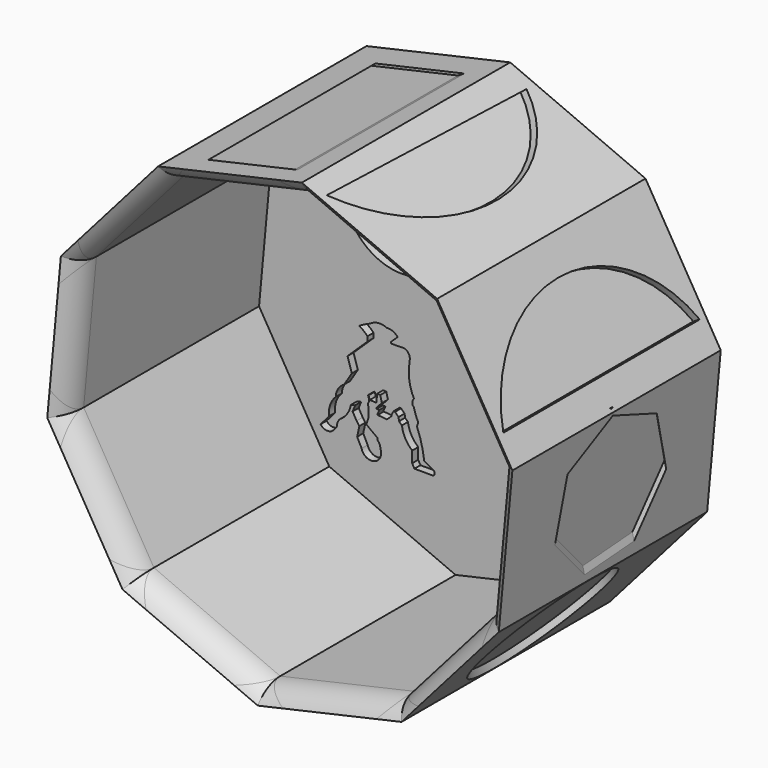
from build123d import *

# Parameters (mm, degrees)
F1_DEPTH      = 25.4
F1_DEPTH_BACK = 12.7
F2_DEPTH      = 19.05
F3_T          = -2.54
F4_T4_DEPTH   = 48.5082887961
F4_T10_DEPTH  = 48.5082887961
F4_T16_DEPTH  = 48.5082887961
F4_T22_DEPTH  = 48.5082887961
F4_T28_DEPTH  = 48.5082887961
F4_T34_DEPTH  = 48.5082887961
F4_T40_DEPTH  = 48.5082887961
F4_T46_DEPTH  = 48.5082887961
F4_T52_DEPTH  = 48.5082887961
F4_T58_DEPTH  = 48.5082887961
F4_T65_DEPTH  = 48.5082887961
F4_T71_DEPTH  = 48.5082887961
F4_T80_DEPTH  = 48.5082887961
F4_T86_DEPTH  = 48.5082887961
F4_T95_DEPTH  = 48.5082887961
F4_T101_DEPTH = 48.5082887961
F4_T110_DEPTH = 48.5082887961
F4_T116_DEPTH = 48.5082887961
F4_T125_DEPTH = 48.5082887961
F4_T131_DEPTH = 48.5082887961
F4_T140_DEPTH = 48.5082887961
F4_T146_DEPTH = 48.5082887961
F4_T155_DEPTH = 48.5082887961
F4_T161_DEPTH = 48.5082887961
F4_T170_DEPTH = 48.5082887961
F4_T176_DEPTH = 48.5082887961
F4_T185_DEPTH = 48.5082887961
F4_T191_DEPTH = 48.5082887961
F4_T200_DEPTH = 48.5082887961
F4_T206_DEPTH = 48.5082887961
F5_R          = 9.7214330453
F5_R_2        = 9.651520044
F6_DEPTH      = 1.27
F8_R          = 12.2677315005
F17_DEPTH     = 1.27
F12_W         = 15.3330643661
F12_H         = 35.0531535223
F18_DEPTH     = 1.27
F19_DEPTH     = 1.27


# Not quite as in the source:
# - a fillet or chamfer that OpenCascade refuses, or shapes differently, is made with other operations: its cross-section is extruded or revolved along the edge and cut away or added


with BuildPart() as f1:
    # F0 (on Front) → F1 (new body, two sides)
    with BuildSketch(Plane.XZ) as f1_sk:
        Polygon((26.439509189, 30.0967257209), (3.6996007358, 39.8895161624), (-20.4534294537, 34.4458672246), (-36.7939447783, 15.845067779), (-39.0804237778, -8.8080090041), (-26.439509189, -30.0967257209), (-3.6996007358, -39.8895161624), (20.4534294537, -34.4458672246), (36.7939447783, -15.845067779), (39.0804237778, 8.8080090041), align=None)
    extrude(amount=F1_DEPTH)
    extrude(f1_sk.sketch, amount=-F1_DEPTH_BACK)

    # F0 (on Front) → F2 (join)
    with BuildSketch(Plane.XZ):
        Polygon((26.439509189, 30.0967257209), (3.6996007358, 39.8895161624), (-20.4534294537, 34.4458672246), (-36.7939447783, 15.845067779), (-39.0804237778, -8.8080090041), (-26.439509189, -30.0967257209), (-3.6996007358, -39.8895161624), (20.4534294537, -34.4458672246), (36.7939447783, -15.845067779), (39.0804237778, 8.8080090041), align=None)
    extrude(amount=-F2_DEPTH)

    # F3
    f3_openings = [f1.faces().sort_by_distance(p)[0] for p in [
        (0, -25.4, 0),
    ]]
    offset(amount=F3_T, openings=f3_openings)

    # F4: fillet of radius 5.08 on 10 edges, made by hand


with BuildPart() as f4_tool2:
    # F4_s3 → F4_t4 (new body)
    with BuildSketch(Plane(origin=(12.383215929, 0, -20.8547232956), x_dir=(0, 1, 0), z_dir=(-0.5105608232, 0, 0.85984164))):
        with BuildLine():
            ThreePointArc((-25.4, -40.64), (-23.9121024484, -37.0478975516), (-20.32, -35.56))
            Line((-20.32, -35.56), (-25.4, -35.56))
            Line((-25.4, -35.56), (-25.4, -40.64))
        make_face()
    extrude(amount=F4_T4_DEPTH)

    split(bisect_by=Plane(origin=(35.4080386595, 0, -3.2839607616), x_dir=(0, 1, 0), z_dir=(-0.9957266215, 0, 0.0923498527)), keep=Keep.TOP)

    split(bisect_by=Plane(origin=(14.0649179649, 0, 32.6602462122), x_dir=(0, 1, 0), z_dir=(-0.395526377, 0, -0.9184546179)), keep=Keep.TOP)


with BuildPart() as f1_1:
    add(f1.part)

    # F4_t1: cut F4_tool2
    add(f4_tool2.part, mode=Mode.SUBTRACT)


with BuildPart() as f4_tool8:
    # F4_s9 → F4_t10 (new body)
    with BuildSketch(Plane(origin=(-2.2398666623, 0, -24.1504972582), x_dir=(0, 1, 0), z_dir=(0.0923498527, 0, 0.9957266215))):
        with BuildLine():
            ThreePointArc((-25.4, -40.64), (-23.9121024484, -37.0478975516), (-20.32, -35.56))
            Line((-20.32, -35.56), (-25.4, -35.56))
            Line((-25.4, -35.56), (-25.4, -40.64))
        make_face()
    extrude(amount=F4_T10_DEPTH)

    split(bisect_by=Plane(origin=(30.5759687179, 0, 18.1555428717), x_dir=(0, 1, 0), z_dir=(-0.85984164, 0, -0.5105608232)), keep=Keep.TOP)

    split(bisect_by=Plane(origin=(26.7154413083, 0, -23.4691030017), x_dir=(0, 1, 0), z_dir=(-0.7512778771, 0, 0.6599860237)), keep=Keep.TOP)


with BuildPart() as f1_2:
    add(f1_1.part)

    # F4_t7: cut F4_tool8
    add(f4_tool8.part, mode=Mode.SUBTRACT)


with BuildPart() as f4_tool14:
    # F4_s15 → F4_t16 (new body)
    with BuildSketch(Plane(origin=(-16.0073963188, 0, -18.2216021133), x_dir=(0, 1, 0), z_dir=(0.6599860237, 0, 0.7512778771))):
        with BuildLine():
            ThreePointArc((-25.4, -40.64), (-23.9121024484, -37.0478975516), (-20.32, -35.56))
            Line((-20.32, -35.56), (-25.4, -35.56))
            Line((-25.4, -35.56), (-25.4, -40.64))
        make_face()
    extrude(amount=F4_T16_DEPTH)

    split(bisect_by=Plane(origin=(35.4080386595, 0, -3.2839607616), x_dir=(0, 1, 0), z_dir=(-0.9957266215, 0, 0.0923498527)), keep=Keep.TOP)

    split(bisect_by=Plane(origin=(7.8184534017, 0, -34.6898455806), x_dir=(0, 1, 0), z_dir=(-0.2198665186, 0, 0.9755299657)), keep=Keep.TOP)


with BuildPart() as f1_3:
    add(f1_2.part)

    # F4_t13: cut F4_tool14
    add(f4_tool14.part, mode=Mode.SUBTRACT)


with BuildPart() as f4_tool20:
    # F4_s21 → F4_t22 (new body)
    with BuildSketch(Plane(origin=(-23.6606446529, 0, -5.3326742906), x_dir=(0, 1, 0), z_dir=(0.9755299657, 0, 0.2198665186))):
        with BuildLine():
            ThreePointArc((-25.4, -40.64), (-23.9121024484, -37.0478975516), (-20.32, -35.56))
            Line((-20.32, -35.56), (-25.4, -35.56))
            Line((-25.4, -35.56), (-25.4, -40.64))
        make_face()
    extrude(amount=F4_T22_DEPTH)

    split(bisect_by=Plane(origin=(-14.0649179649, 0, -32.6602462122), x_dir=(0, 1, 0), z_dir=(0.395526377, 0, 0.9184546179)), keep=Keep.TOP)

    split(bisect_by=Plane(origin=(26.7154413083, 0, -23.4691030017), x_dir=(0, 1, 0), z_dir=(-0.7512778771, 0, 0.6599860237)), keep=Keep.TOP)


with BuildPart() as f1_4:
    add(f1_3.part)

    # F4_t19: cut F4_tool20
    add(f4_tool20.part, mode=Mode.SUBTRACT)


with BuildPart() as f4_tool26:
    # F4_s27 → F4_t28 (new body)
    with BuildSketch(Plane(origin=(-22.2763309254, 0, 9.5931538602), x_dir=(0, 1, 0), z_dir=(0.9184546179, 0, -0.395526377))):
        with BuildLine():
            ThreePointArc((-25.4, -40.64), (-23.9121024484, -37.0478975516), (-20.32, -35.56))
            Line((-20.32, -35.56), (-25.4, -35.56))
            Line((-25.4, -35.56), (-25.4, -40.64))
        make_face()
    extrude(amount=F4_T28_DEPTH)

    split(bisect_by=Plane(origin=(-30.5759687179, 0, -18.1555428717), x_dir=(0, 1, 0), z_dir=(0.85984164, 0, 0.5105608232)), keep=Keep.TOP)

    split(bisect_by=Plane(origin=(7.8184534017, 0, -34.6898455806), x_dir=(0, 1, 0), z_dir=(-0.2198665186, 0, 0.9755299657)), keep=Keep.TOP)


with BuildPart() as f1_5:
    add(f1_4.part)

    # F4_t25: cut F4_tool26
    add(f4_tool26.part, mode=Mode.SUBTRACT)


with BuildPart() as f4_tool32:
    # F4_s33 → F4_t34 (new body)
    with BuildSketch(Plane(origin=(22.2763309254, 0, -9.5931538602), x_dir=(0, 1, 0), z_dir=(-0.9184546179, 0, 0.395526377))):
        with BuildLine():
            ThreePointArc((-25.4, -40.64), (-23.9121024484, -37.0478975516), (-20.32, -35.56))
            Line((-20.32, -35.56), (-25.4, -35.56))
            Line((-25.4, -35.56), (-25.4, -40.64))
        make_face()
    extrude(amount=F4_T34_DEPTH)

    split(bisect_by=Plane(origin=(30.5759687179, 0, 18.1555428717), x_dir=(0, 1, 0), z_dir=(-0.85984164, 0, -0.5105608232)), keep=Keep.TOP)

    split(bisect_by=Plane(origin=(-7.8184534017, 0, 34.6898455806), x_dir=(0, 1, 0), z_dir=(0.2198665186, 0, -0.9755299657)), keep=Keep.TOP)


with BuildPart() as f1_6:
    add(f1_5.part)

    # F4_t31: cut F4_tool32
    add(f4_tool32.part, mode=Mode.SUBTRACT)


with BuildPart() as f4_tool38:
    # F4_s39 → F4_t40 (new body)
    with BuildSketch(Plane(origin=(23.6606446529, 0, 5.3326742906), x_dir=(0, 1, 0), z_dir=(-0.9755299657, 0, -0.2198665186))):
        with BuildLine():
            ThreePointArc((-25.4, -40.64), (-23.9121024484, -37.0478975516), (-20.32, -35.56))
            Line((-20.32, -35.56), (-25.4, -35.56))
            Line((-25.4, -35.56), (-25.4, -40.64))
        make_face()
    extrude(amount=F4_T40_DEPTH)

    split(bisect_by=Plane(origin=(14.0649179649, 0, 32.6602462122), x_dir=(0, 1, 0), z_dir=(-0.395526377, 0, -0.9184546179)), keep=Keep.TOP)

    split(bisect_by=Plane(origin=(-26.7154413083, 0, 23.4691030017), x_dir=(0, 1, 0), z_dir=(0.7512778771, 0, -0.6599860237)), keep=Keep.TOP)


with BuildPart() as f1_7:
    add(f1_6.part)

    # F4_t37: cut F4_tool38
    add(f4_tool38.part, mode=Mode.SUBTRACT)


with BuildPart() as f4_tool44:
    # F4_s45 → F4_t46 (new body)
    with BuildSketch(Plane(origin=(16.0073963188, 0, 18.2216021133), x_dir=(0, 1, 0), z_dir=(-0.6599860237, 0, -0.7512778771))):
        with BuildLine():
            ThreePointArc((-25.4, -40.64), (-23.9121024484, -37.0478975516), (-20.32, -35.56))
            Line((-20.32, -35.56), (-25.4, -35.56))
            Line((-25.4, -35.56), (-25.4, -40.64))
        make_face()
    extrude(amount=F4_T46_DEPTH)

    split(bisect_by=Plane(origin=(-7.8184534017, 0, 34.6898455806), x_dir=(0, 1, 0), z_dir=(0.2198665186, 0, -0.9755299657)), keep=Keep.TOP)

    split(bisect_by=Plane(origin=(-35.4080386595, 0, 3.2839607616), x_dir=(0, 1, 0), z_dir=(0.9957266215, 0, -0.0923498527)), keep=Keep.TOP)


with BuildPart() as f1_8:
    add(f1_7.part)

    # F4_t43: cut F4_tool44
    add(f4_tool44.part, mode=Mode.SUBTRACT)


with BuildPart() as f4_tool50:
    # F4_s51 → F4_t52 (new body)
    with BuildSketch(Plane(origin=(2.2398666623, 0, 24.1504972582), x_dir=(0, 1, 0), z_dir=(-0.0923498527, 0, -0.9957266215))):
        with BuildLine():
            ThreePointArc((-25.4, -40.64), (-23.9121024484, -37.0478975516), (-20.32, -35.56))
            Line((-20.32, -35.56), (-25.4, -35.56))
            Line((-25.4, -35.56), (-25.4, -40.64))
        make_face()
    extrude(amount=F4_T52_DEPTH)

    split(bisect_by=Plane(origin=(-26.7154413083, 0, 23.4691030017), x_dir=(0, 1, 0), z_dir=(0.7512778771, 0, -0.6599860237)), keep=Keep.TOP)

    split(bisect_by=Plane(origin=(-30.5759687179, 0, -18.1555428717), x_dir=(0, 1, 0), z_dir=(0.85984164, 0, 0.5105608232)), keep=Keep.TOP)


with BuildPart() as f1_9:
    add(f1_8.part)

    # F4_t49: cut F4_tool50
    add(f4_tool50.part, mode=Mode.SUBTRACT)


with BuildPart() as f4_tool56:
    # F4_s57 → F4_t58 (new body)
    with BuildSketch(Plane(origin=(-12.383215929, 0, 20.8547232956), x_dir=(0, 1, 0), z_dir=(0.5105608232, 0, -0.85984164))):
        with BuildLine():
            ThreePointArc((-25.4, -40.64), (-23.9121024484, -37.0478975516), (-20.32, -35.56))
            Line((-20.32, -35.56), (-25.4, -35.56))
            Line((-25.4, -35.56), (-25.4, -40.64))
        make_face()
    extrude(amount=F4_T58_DEPTH)

    split(bisect_by=Plane(origin=(-35.4080386595, 0, 3.2839607616), x_dir=(0, 1, 0), z_dir=(0.9957266215, 0, -0.0923498527)), keep=Keep.TOP)

    split(bisect_by=Plane(origin=(-14.0649179649, 0, -32.6602462122), x_dir=(0, 1, 0), z_dir=(0.395526377, 0, 0.9184546179)), keep=Keep.TOP)


with BuildPart() as f1_10:
    add(f1_9.part)

    # F4_t55: cut F4_tool56
    add(f4_tool56.part, mode=Mode.SUBTRACT)


with BuildPart() as f4_tool63:
    # F4_s64 → F4_t65 (new body)
    with BuildSketch(Plane(origin=(-2.2398666623, 0, -24.1504972582), x_dir=(0, 1, 0), z_dir=(0.0923498527, 0, 0.9957266215))):
        with BuildLine():
            ThreePointArc((-25.4, -40.64), (-23.9121024484, -37.0478975516), (-20.32, -35.56))
            Line((-20.32, -35.56), (-25.4, -35.56))
            Line((-25.4, -35.56), (-25.4, -40.64))
        make_face()
    extrude(amount=F4_T65_DEPTH)

    split(bisect_by=Plane(origin=(37.9371842781, 0, -3.5185293875), x_dir=(0, 1, 0), z_dir=(-0.9957266215, 0, 0.0923498527)), keep=Keep.TOP)

    split(bisect_by=Plane(origin=(32.7599664834, 0, 19.4523673625), x_dir=(0, 1, 0), z_dir=(-0.85984164, 0, -0.5105608232)), keep=Keep.TOP)

    split(bisect_by=Plane(origin=(30.5759687179, 0, 18.1555428717), x_dir=(0, 1, 0), z_dir=(0.85984164, 0, 0.5105608232)), keep=Keep.TOP)


with BuildPart() as f4_tool69:
    # F4_s70 → F4_t71 (new body)
    with BuildSketch(Plane(origin=(12.383215929, 0, -20.8547232956), x_dir=(0, 1, 0), z_dir=(-0.5105608232, 0, 0.85984164))):
        with BuildLine():
            ThreePointArc((-25.4, -40.64), (-23.9121024484, -37.0478975516), (-20.32, -35.56))
            Line((-20.32, -35.56), (-25.4, -35.56))
            Line((-25.4, -35.56), (-25.4, -40.64))
        make_face()
    extrude(amount=F4_T71_DEPTH)

    split(bisect_by=Plane(origin=(37.9371842781, 0, -3.5185293875), x_dir=(0, 1, 0), z_dir=(-0.9957266215, 0, 0.0923498527)), keep=Keep.TOP)

    split(bisect_by=Plane(origin=(32.7599664834, 0, 19.4523673625), x_dir=(0, 1, 0), z_dir=(-0.85984164, 0, -0.5105608232)), keep=Keep.TOP)

    split(bisect_by=Plane(origin=(35.4080386595, 0, -3.2839607616), x_dir=(0, 1, 0), z_dir=(0.9957266215, 0, -0.0923498527)), keep=Keep.TOP)


with BuildPart() as f4_tool63_1:
    add(f4_tool63.part)

    # F4_t75: intersect F4_tool69
    add(f4_tool69.part, mode=Mode.INTERSECT)


with BuildPart() as f1_11:
    add(f1_10.part)

    # F4_t61: cut F4_tool63
    add(f4_tool63_1.part, mode=Mode.SUBTRACT)


with BuildPart() as f4_tool78:
    # F4_s79 → F4_t80 (new body)
    with BuildSketch(Plane(origin=(22.2763309254, 0, -9.5931538602), x_dir=(0, 1, 0), z_dir=(-0.9184546179, 0, 0.395526377))):
        with BuildLine():
            ThreePointArc((-25.4, -40.64), (-23.9121024484, -37.0478975516), (-20.32, -35.56))
            Line((-20.32, -35.56), (-25.4, -35.56))
            Line((-25.4, -35.56), (-25.4, -40.64))
        make_face()
    extrude(amount=F4_T80_DEPTH)

    split(bisect_by=Plane(origin=(15.0695549624, 0, 34.9931209416), x_dir=(0, 1, 0), z_dir=(-0.395526377, 0, -0.9184546179)), keep=Keep.TOP)

    split(bisect_by=Plane(origin=(32.7599664834, 0, 19.4523673625), x_dir=(0, 1, 0), z_dir=(-0.85984164, 0, -0.5105608232)), keep=Keep.TOP)

    split(bisect_by=Plane(origin=(30.5759687179, 0, 18.1555428717), x_dir=(0, 1, 0), z_dir=(0.85984164, 0, 0.5105608232)), keep=Keep.TOP)


with BuildPart() as f4_tool84:
    # F4_s85 → F4_t86 (new body)
    with BuildSketch(Plane(origin=(12.383215929, 0, -20.8547232956), x_dir=(0, 1, 0), z_dir=(-0.5105608232, 0, 0.85984164))):
        with BuildLine():
            ThreePointArc((-25.4, -40.64), (-23.9121024484, -37.0478975516), (-20.32, -35.56))
            Line((-20.32, -35.56), (-25.4, -35.56))
            Line((-25.4, -35.56), (-25.4, -40.64))
        make_face()
    extrude(amount=F4_T86_DEPTH)

    split(bisect_by=Plane(origin=(15.0695549624, 0, 34.9931209416), x_dir=(0, 1, 0), z_dir=(-0.395526377, 0, -0.9184546179)), keep=Keep.TOP)

    split(bisect_by=Plane(origin=(32.7599664834, 0, 19.4523673625), x_dir=(0, 1, 0), z_dir=(-0.85984164, 0, -0.5105608232)), keep=Keep.TOP)

    split(bisect_by=Plane(origin=(14.0649179649, 0, 32.6602462122), x_dir=(0, 1, 0), z_dir=(0.395526377, 0, 0.9184546179)), keep=Keep.TOP)


with BuildPart() as f4_tool78_1:
    add(f4_tool78.part)

    # F4_t90: intersect F4_tool84
    add(f4_tool84.part, mode=Mode.INTERSECT)


with BuildPart() as f1_12:
    add(f1_11.part)

    # F4_t76: cut F4_tool78
    add(f4_tool78_1.part, mode=Mode.SUBTRACT)


with BuildPart() as f4_tool93:
    # F4_s94 → F4_t95 (new body)
    with BuildSketch(Plane(origin=(-2.2398666623, 0, -24.1504972582), x_dir=(0, 1, 0), z_dir=(0.0923498527, 0, 0.9957266215))):
        with BuildLine():
            ThreePointArc((-25.4, -40.64), (-23.9121024484, -37.0478975516), (-20.32, -35.56))
            Line((-20.32, -35.56), (-25.4, -35.56))
            Line((-25.4, -35.56), (-25.4, -40.64))
        make_face()
    extrude(amount=F4_T95_DEPTH)

    split(bisect_by=Plane(origin=(37.9371842781, 0, -3.5185293875), x_dir=(0, 1, 0), z_dir=(-0.9957266215, 0, 0.0923498527)), keep=Keep.TOP)

    split(bisect_by=Plane(origin=(28.623687116, 0, -25.1454675018), x_dir=(0, 1, 0), z_dir=(-0.7512778771, 0, 0.6599860237)), keep=Keep.TOP)

    split(bisect_by=Plane(origin=(26.7154413083, 0, -23.4691030017), x_dir=(0, 1, 0), z_dir=(0.7512778771, 0, -0.6599860237)), keep=Keep.TOP)


with BuildPart() as f4_tool99:
    # F4_s100 → F4_t101 (new body)
    with BuildSketch(Plane(origin=(-16.0073963188, 0, -18.2216021133), x_dir=(0, 1, 0), z_dir=(0.6599860237, 0, 0.7512778771))):
        with BuildLine():
            ThreePointArc((-25.4, -40.64), (-23.9121024484, -37.0478975516), (-20.32, -35.56))
            Line((-20.32, -35.56), (-25.4, -35.56))
            Line((-25.4, -35.56), (-25.4, -40.64))
        make_face()
    extrude(amount=F4_T101_DEPTH)

    split(bisect_by=Plane(origin=(37.9371842781, 0, -3.5185293875), x_dir=(0, 1, 0), z_dir=(-0.9957266215, 0, 0.0923498527)), keep=Keep.TOP)

    split(bisect_by=Plane(origin=(28.623687116, 0, -25.1454675018), x_dir=(0, 1, 0), z_dir=(-0.7512778771, 0, 0.6599860237)), keep=Keep.TOP)

    split(bisect_by=Plane(origin=(35.4080386595, 0, -3.2839607616), x_dir=(0, 1, 0), z_dir=(0.9957266215, 0, -0.0923498527)), keep=Keep.TOP)


with BuildPart() as f4_tool93_1:
    add(f4_tool93.part)

    # F4_t105: intersect F4_tool99
    add(f4_tool99.part, mode=Mode.INTERSECT)


with BuildPart() as f1_13:
    add(f1_12.part)

    # F4_t91: cut F4_tool93
    add(f4_tool93_1.part, mode=Mode.SUBTRACT)


with BuildPart() as f4_tool108:
    # F4_s109 → F4_t110 (new body)
    with BuildSketch(Plane(origin=(-16.0073963188, 0, -18.2216021133), x_dir=(0, 1, 0), z_dir=(0.6599860237, 0, 0.7512778771))):
        with BuildLine():
            ThreePointArc((-25.4, -40.64), (-23.9121024484, -37.0478975516), (-20.32, -35.56))
            Line((-20.32, -35.56), (-25.4, -35.56))
            Line((-25.4, -35.56), (-25.4, -40.64))
        make_face()
    extrude(amount=F4_T110_DEPTH)

    split(bisect_by=Plane(origin=(8.3769143589, 0, -37.1676916935), x_dir=(0, 1, 0), z_dir=(-0.2198665186, 0, 0.9755299657)), keep=Keep.TOP)

    split(bisect_by=Plane(origin=(28.623687116, 0, -25.1454675018), x_dir=(0, 1, 0), z_dir=(-0.7512778771, 0, 0.6599860237)), keep=Keep.TOP)

    split(bisect_by=Plane(origin=(7.8184534017, 0, -34.6898455806), x_dir=(0, 1, 0), z_dir=(0.2198665186, 0, -0.9755299657)), keep=Keep.TOP)


with BuildPart() as f4_tool114:
    # F4_s115 → F4_t116 (new body)
    with BuildSketch(Plane(origin=(-23.6606446529, 0, -5.3326742906), x_dir=(0, 1, 0), z_dir=(0.9755299657, 0, 0.2198665186))):
        with BuildLine():
            ThreePointArc((-25.4, -40.64), (-23.9121024484, -37.0478975516), (-20.32, -35.56))
            Line((-20.32, -35.56), (-25.4, -35.56))
            Line((-25.4, -35.56), (-25.4, -40.64))
        make_face()
    extrude(amount=F4_T116_DEPTH)

    split(bisect_by=Plane(origin=(8.3769143589, 0, -37.1676916935), x_dir=(0, 1, 0), z_dir=(-0.2198665186, 0, 0.9755299657)), keep=Keep.TOP)

    split(bisect_by=Plane(origin=(28.623687116, 0, -25.1454675018), x_dir=(0, 1, 0), z_dir=(-0.7512778771, 0, 0.6599860237)), keep=Keep.TOP)

    split(bisect_by=Plane(origin=(26.7154413083, 0, -23.4691030017), x_dir=(0, 1, 0), z_dir=(0.7512778771, 0, -0.6599860237)), keep=Keep.TOP)


with BuildPart() as f4_tool108_1:
    add(f4_tool108.part)

    # F4_t120: intersect F4_tool114
    add(f4_tool114.part, mode=Mode.INTERSECT)


with BuildPart() as f1_14:
    add(f1_13.part)

    # F4_t106: cut F4_tool108
    add(f4_tool108_1.part, mode=Mode.SUBTRACT)


with BuildPart() as f4_tool123:
    # F4_s124 → F4_t125 (new body)
    with BuildSketch(Plane(origin=(-23.6606446529, 0, -5.3326742906), x_dir=(0, 1, 0), z_dir=(0.9755299657, 0, 0.2198665186))):
        with BuildLine():
            ThreePointArc((-25.4, -40.64), (-23.9121024484, -37.0478975516), (-20.32, -35.56))
            Line((-20.32, -35.56), (-25.4, -35.56))
            Line((-25.4, -35.56), (-25.4, -40.64))
        make_face()
    extrude(amount=F4_T125_DEPTH)

    split(bisect_by=Plane(origin=(8.3769143589, 0, -37.1676916935), x_dir=(0, 1, 0), z_dir=(-0.2198665186, 0, 0.9755299657)), keep=Keep.TOP)

    split(bisect_by=Plane(origin=(-15.0695549624, 0, -34.9931209416), x_dir=(0, 1, 0), z_dir=(0.395526377, 0, 0.9184546179)), keep=Keep.TOP)

    split(bisect_by=Plane(origin=(-14.0649179649, 0, -32.6602462122), x_dir=(0, 1, 0), z_dir=(-0.395526377, 0, -0.9184546179)), keep=Keep.TOP)


with BuildPart() as f4_tool129:
    # F4_s130 → F4_t131 (new body)
    with BuildSketch(Plane(origin=(-22.2763309254, 0, 9.5931538602), x_dir=(0, 1, 0), z_dir=(0.9184546179, 0, -0.395526377))):
        with BuildLine():
            ThreePointArc((-25.4, -40.64), (-23.9121024484, -37.0478975516), (-20.32, -35.56))
            Line((-20.32, -35.56), (-25.4, -35.56))
            Line((-25.4, -35.56), (-25.4, -40.64))
        make_face()
    extrude(amount=F4_T131_DEPTH)

    split(bisect_by=Plane(origin=(8.3769143589, 0, -37.1676916935), x_dir=(0, 1, 0), z_dir=(-0.2198665186, 0, 0.9755299657)), keep=Keep.TOP)

    split(bisect_by=Plane(origin=(-15.0695549624, 0, -34.9931209416), x_dir=(0, 1, 0), z_dir=(0.395526377, 0, 0.9184546179)), keep=Keep.TOP)

    split(bisect_by=Plane(origin=(7.8184534017, 0, -34.6898455806), x_dir=(0, 1, 0), z_dir=(0.2198665186, 0, -0.9755299657)), keep=Keep.TOP)


with BuildPart() as f4_tool123_1:
    add(f4_tool123.part)

    # F4_t135: intersect F4_tool129
    add(f4_tool129.part, mode=Mode.INTERSECT)


with BuildPart() as f1_15:
    add(f1_14.part)

    # F4_t121: cut F4_tool123
    add(f4_tool123_1.part, mode=Mode.SUBTRACT)


with BuildPart() as f4_tool138:
    # F4_s139 → F4_t140 (new body)
    with BuildSketch(Plane(origin=(-22.2763309254, 0, 9.5931538602), x_dir=(0, 1, 0), z_dir=(0.9184546179, 0, -0.395526377))):
        with BuildLine():
            ThreePointArc((-25.4, -40.64), (-23.9121024484, -37.0478975516), (-20.32, -35.56))
            Line((-20.32, -35.56), (-25.4, -35.56))
            Line((-25.4, -35.56), (-25.4, -40.64))
        make_face()
    extrude(amount=F4_T140_DEPTH)

    split(bisect_by=Plane(origin=(-15.0695549624, 0, -34.9931209416), x_dir=(0, 1, 0), z_dir=(0.395526377, 0, 0.9184546179)), keep=Keep.TOP)

    split(bisect_by=Plane(origin=(-32.7599664834, 0, -19.4523673625), x_dir=(0, 1, 0), z_dir=(0.85984164, 0, 0.5105608232)), keep=Keep.TOP)

    split(bisect_by=Plane(origin=(-30.5759687179, 0, -18.1555428717), x_dir=(0, 1, 0), z_dir=(-0.85984164, 0, -0.5105608232)), keep=Keep.TOP)


with BuildPart() as f4_tool144:
    # F4_s145 → F4_t146 (new body)
    with BuildSketch(Plane(origin=(-12.383215929, 0, 20.8547232956), x_dir=(0, 1, 0), z_dir=(0.5105608232, 0, -0.85984164))):
        with BuildLine():
            ThreePointArc((-25.4, -40.64), (-23.9121024484, -37.0478975516), (-20.32, -35.56))
            Line((-20.32, -35.56), (-25.4, -35.56))
            Line((-25.4, -35.56), (-25.4, -40.64))
        make_face()
    extrude(amount=F4_T146_DEPTH)

    split(bisect_by=Plane(origin=(-15.0695549624, 0, -34.9931209416), x_dir=(0, 1, 0), z_dir=(0.395526377, 0, 0.9184546179)), keep=Keep.TOP)

    split(bisect_by=Plane(origin=(-32.7599664834, 0, -19.4523673625), x_dir=(0, 1, 0), z_dir=(0.85984164, 0, 0.5105608232)), keep=Keep.TOP)

    split(bisect_by=Plane(origin=(-14.0649179649, 0, -32.6602462122), x_dir=(0, 1, 0), z_dir=(-0.395526377, 0, -0.9184546179)), keep=Keep.TOP)


with BuildPart() as f4_tool138_1:
    add(f4_tool138.part)

    # F4_t150: intersect F4_tool144
    add(f4_tool144.part, mode=Mode.INTERSECT)


with BuildPart() as f1_16:
    add(f1_15.part)

    # F4_t136: cut F4_tool138
    add(f4_tool138_1.part, mode=Mode.SUBTRACT)


with BuildPart() as f4_tool153:
    # F4_s154 → F4_t155 (new body)
    with BuildSketch(Plane(origin=(23.6606446529, 0, 5.3326742906), x_dir=(0, 1, 0), z_dir=(-0.9755299657, 0, -0.2198665186))):
        with BuildLine():
            ThreePointArc((-25.4, -40.64), (-23.9121024484, -37.0478975516), (-20.32, -35.56))
            Line((-20.32, -35.56), (-25.4, -35.56))
            Line((-25.4, -35.56), (-25.4, -40.64))
        make_face()
    extrude(amount=F4_T155_DEPTH)

    split(bisect_by=Plane(origin=(-8.3769143589, 0, 37.1676916935), x_dir=(0, 1, 0), z_dir=(0.2198665186, 0, -0.9755299657)), keep=Keep.TOP)

    split(bisect_by=Plane(origin=(15.0695549624, 0, 34.9931209416), x_dir=(0, 1, 0), z_dir=(-0.395526377, 0, -0.9184546179)), keep=Keep.TOP)

    split(bisect_by=Plane(origin=(14.0649179649, 0, 32.6602462122), x_dir=(0, 1, 0), z_dir=(0.395526377, 0, 0.9184546179)), keep=Keep.TOP)


with BuildPart() as f4_tool159:
    # F4_s160 → F4_t161 (new body)
    with BuildSketch(Plane(origin=(22.2763309254, 0, -9.5931538602), x_dir=(0, 1, 0), z_dir=(-0.9184546179, 0, 0.395526377))):
        with BuildLine():
            ThreePointArc((-25.4, -40.64), (-23.9121024484, -37.0478975516), (-20.32, -35.56))
            Line((-20.32, -35.56), (-25.4, -35.56))
            Line((-25.4, -35.56), (-25.4, -40.64))
        make_face()
    extrude(amount=F4_T161_DEPTH)

    split(bisect_by=Plane(origin=(-8.3769143589, 0, 37.1676916935), x_dir=(0, 1, 0), z_dir=(0.2198665186, 0, -0.9755299657)), keep=Keep.TOP)

    split(bisect_by=Plane(origin=(15.0695549624, 0, 34.9931209416), x_dir=(0, 1, 0), z_dir=(-0.395526377, 0, -0.9184546179)), keep=Keep.TOP)

    split(bisect_by=Plane(origin=(-7.8184534017, 0, 34.6898455806), x_dir=(0, 1, 0), z_dir=(-0.2198665186, 0, 0.9755299657)), keep=Keep.TOP)


with BuildPart() as f4_tool153_1:
    add(f4_tool153.part)

    # F4_t165: intersect F4_tool159
    add(f4_tool159.part, mode=Mode.INTERSECT)


with BuildPart() as f1_17:
    add(f1_16.part)

    # F4_t151: cut F4_tool153
    add(f4_tool153_1.part, mode=Mode.SUBTRACT)


with BuildPart() as f4_tool168:
    # F4_s169 → F4_t170 (new body)
    with BuildSketch(Plane(origin=(16.0073963188, 0, 18.2216021133), x_dir=(0, 1, 0), z_dir=(-0.6599860237, 0, -0.7512778771))):
        with BuildLine():
            ThreePointArc((-25.4, -40.64), (-23.9121024484, -37.0478975516), (-20.32, -35.56))
            Line((-20.32, -35.56), (-25.4, -35.56))
            Line((-25.4, -35.56), (-25.4, -40.64))
        make_face()
    extrude(amount=F4_T170_DEPTH)

    split(bisect_by=Plane(origin=(-28.623687116, 0, 25.1454675018), x_dir=(0, 1, 0), z_dir=(0.7512778771, 0, -0.6599860237)), keep=Keep.TOP)

    split(bisect_by=Plane(origin=(-8.3769143589, 0, 37.1676916935), x_dir=(0, 1, 0), z_dir=(0.2198665186, 0, -0.9755299657)), keep=Keep.TOP)

    split(bisect_by=Plane(origin=(-7.8184534017, 0, 34.6898455806), x_dir=(0, 1, 0), z_dir=(-0.2198665186, 0, 0.9755299657)), keep=Keep.TOP)


with BuildPart() as f4_tool174:
    # F4_s175 → F4_t176 (new body)
    with BuildSketch(Plane(origin=(23.6606446529, 0, 5.3326742906), x_dir=(0, 1, 0), z_dir=(-0.9755299657, 0, -0.2198665186))):
        with BuildLine():
            ThreePointArc((-25.4, -40.64), (-23.9121024484, -37.0478975516), (-20.32, -35.56))
            Line((-20.32, -35.56), (-25.4, -35.56))
            Line((-25.4, -35.56), (-25.4, -40.64))
        make_face()
    extrude(amount=F4_T176_DEPTH)

    split(bisect_by=Plane(origin=(-28.623687116, 0, 25.1454675018), x_dir=(0, 1, 0), z_dir=(0.7512778771, 0, -0.6599860237)), keep=Keep.TOP)

    split(bisect_by=Plane(origin=(-8.3769143589, 0, 37.1676916935), x_dir=(0, 1, 0), z_dir=(0.2198665186, 0, -0.9755299657)), keep=Keep.TOP)

    split(bisect_by=Plane(origin=(-26.7154413083, 0, 23.4691030017), x_dir=(0, 1, 0), z_dir=(-0.7512778771, 0, 0.6599860237)), keep=Keep.TOP)


with BuildPart() as f4_tool168_1:
    add(f4_tool168.part)

    # F4_t180: intersect F4_tool174
    add(f4_tool174.part, mode=Mode.INTERSECT)


with BuildPart() as f1_18:
    add(f1_17.part)

    # F4_t166: cut F4_tool168
    add(f4_tool168_1.part, mode=Mode.SUBTRACT)


with BuildPart() as f4_tool183:
    # F4_s184 → F4_t185 (new body)
    with BuildSketch(Plane(origin=(2.2398666623, 0, 24.1504972582), x_dir=(0, 1, 0), z_dir=(-0.0923498527, 0, -0.9957266215))):
        with BuildLine():
            ThreePointArc((-25.4, -40.64), (-23.9121024484, -37.0478975516), (-20.32, -35.56))
            Line((-20.32, -35.56), (-25.4, -35.56))
            Line((-25.4, -35.56), (-25.4, -40.64))
        make_face()
    extrude(amount=F4_T185_DEPTH)

    split(bisect_by=Plane(origin=(-37.9371842781, 0, 3.5185293875), x_dir=(0, 1, 0), z_dir=(0.9957266215, 0, -0.0923498527)), keep=Keep.TOP)

    split(bisect_by=Plane(origin=(-28.623687116, 0, 25.1454675018), x_dir=(0, 1, 0), z_dir=(0.7512778771, 0, -0.6599860237)), keep=Keep.TOP)

    split(bisect_by=Plane(origin=(-26.7154413083, 0, 23.4691030017), x_dir=(0, 1, 0), z_dir=(-0.7512778771, 0, 0.6599860237)), keep=Keep.TOP)


with BuildPart() as f4_tool189:
    # F4_s190 → F4_t191 (new body)
    with BuildSketch(Plane(origin=(16.0073963188, 0, 18.2216021133), x_dir=(0, 1, 0), z_dir=(-0.6599860237, 0, -0.7512778771))):
        with BuildLine():
            ThreePointArc((-25.4, -40.64), (-23.9121024484, -37.0478975516), (-20.32, -35.56))
            Line((-20.32, -35.56), (-25.4, -35.56))
            Line((-25.4, -35.56), (-25.4, -40.64))
        make_face()
    extrude(amount=F4_T191_DEPTH)

    split(bisect_by=Plane(origin=(-37.9371842781, 0, 3.5185293875), x_dir=(0, 1, 0), z_dir=(0.9957266215, 0, -0.0923498527)), keep=Keep.TOP)

    split(bisect_by=Plane(origin=(-28.623687116, 0, 25.1454675018), x_dir=(0, 1, 0), z_dir=(0.7512778771, 0, -0.6599860237)), keep=Keep.TOP)

    split(bisect_by=Plane(origin=(-35.4080386595, 0, 3.2839607616), x_dir=(0, 1, 0), z_dir=(-0.9957266215, 0, 0.0923498527)), keep=Keep.TOP)


with BuildPart() as f4_tool183_1:
    add(f4_tool183.part)

    # F4_t195: intersect F4_tool189
    add(f4_tool189.part, mode=Mode.INTERSECT)


with BuildPart() as f1_19:
    add(f1_18.part)

    # F4_t181: cut F4_tool183
    add(f4_tool183_1.part, mode=Mode.SUBTRACT)


with BuildPart() as f4_tool198:
    # F4_s199 → F4_t200 (new body)
    with BuildSketch(Plane(origin=(-12.383215929, 0, 20.8547232956), x_dir=(0, 1, 0), z_dir=(0.5105608232, 0, -0.85984164))):
        with BuildLine():
            ThreePointArc((-25.4, -40.64), (-23.9121024484, -37.0478975516), (-20.32, -35.56))
            Line((-20.32, -35.56), (-25.4, -35.56))
            Line((-25.4, -35.56), (-25.4, -40.64))
        make_face()
    extrude(amount=F4_T200_DEPTH)

    split(bisect_by=Plane(origin=(-32.7599664834, 0, -19.4523673625), x_dir=(0, 1, 0), z_dir=(0.85984164, 0, 0.5105608232)), keep=Keep.TOP)

    split(bisect_by=Plane(origin=(-37.9371842781, 0, 3.5185293875), x_dir=(0, 1, 0), z_dir=(0.9957266215, 0, -0.0923498527)), keep=Keep.TOP)

    split(bisect_by=Plane(origin=(-35.4080386595, 0, 3.2839607616), x_dir=(0, 1, 0), z_dir=(-0.9957266215, 0, 0.0923498527)), keep=Keep.TOP)


with BuildPart() as f4_tool204:
    # F4_s205 → F4_t206 (new body)
    with BuildSketch(Plane(origin=(2.2398666623, 0, 24.1504972582), x_dir=(0, 1, 0), z_dir=(-0.0923498527, 0, -0.9957266215))):
        with BuildLine():
            ThreePointArc((-25.4, -40.64), (-23.9121024484, -37.0478975516), (-20.32, -35.56))
            Line((-20.32, -35.56), (-25.4, -35.56))
            Line((-25.4, -35.56), (-25.4, -40.64))
        make_face()
    extrude(amount=F4_T206_DEPTH)

    split(bisect_by=Plane(origin=(-32.7599664834, 0, -19.4523673625), x_dir=(0, 1, 0), z_dir=(0.85984164, 0, 0.5105608232)), keep=Keep.TOP)

    split(bisect_by=Plane(origin=(-37.9371842781, 0, 3.5185293875), x_dir=(0, 1, 0), z_dir=(0.9957266215, 0, -0.0923498527)), keep=Keep.TOP)

    split(bisect_by=Plane(origin=(-30.5759687179, 0, -18.1555428717), x_dir=(0, 1, 0), z_dir=(-0.85984164, 0, -0.5105608232)), keep=Keep.TOP)


with BuildPart() as f4_tool198_1:
    add(f4_tool198.part)

    # F4_t210: intersect F4_tool204
    add(f4_tool204.part, mode=Mode.INTERSECT)


with BuildPart() as f1_20:
    add(f1_19.part)

    # F4_t196: cut F4_tool198
    add(f4_tool198_1.part, mode=Mode.SUBTRACT)

    # F5 (on face) → F6 (cut)
    with BuildSketch(Plane.XZ.offset(-16.51)):
        with Locations((-12.4513767078, 14.0991013031)):
            Circle(F5_R)
        with BuildLine():
            ThreePointArc((-10.9998071566, 6.21227175), (-12.5347634081, 8.054217186), (-12.958326377, 10.4141850024))
            Line((-12.958326377, 10.4141850024), (-14.5558063372, 8.7227365002))
            ThreePointArc((-14.5558063372, 8.7227365002), (-16.7079940278, 8.4004370916), (-17.5329837948, 10.4141850024))
            ThreePointArc((-17.5329837948, 10.4141850024), (-18.210494601, 12.2814065414), (-16.675055027, 13.5415503755))
            ThreePointArc((-16.675055027, 13.5415503755), (-15.2218390442, 13.4073100926), (-13.8049935922, 13.0574442446))
            ThreePointArc((-13.8049935922, 13.0574442446), (-14.7835016484, 14.3479388098), (-15.2467563748, 15.8997923136))
            ThreePointArc((-15.2467563748, 15.8997923136), (-14.3593816522, 17.405434917), (-12.6329865307, 17.1334911138))
            ThreePointArc((-12.6329865307, 17.1334911138), (-10.7805481379, 17.5419869247), (-9.8310252652, 15.8997923136))
            ThreePointArc((-9.8310252652, 15.8997923136), (-10.2532675184, 14.2458436671), (-11.2424064428, 12.8546431661))
            ThreePointArc((-11.2424064428, 12.8546431661), (-9.7809597532, 13.3520096849), (-8.2408683375, 13.4583972394))
            ThreePointArc((-8.2408683375, 13.4583972394), (-6.8092987103, 12.2460864031), (-7.4566681869, 10.485404171))
            ThreePointArc((-7.4566681869, 10.485404171), (-8.1378352048, 8.5310539925), (-10.1985950023, 8.7227365002))
            Line((-10.1985950023, 8.7227365002), (-12.1215041727, 10.5388183147))
            ThreePointArc((-12.1215041727, 10.5388183147), (-11.8974605138, 8.5988273745), (-10.7327364385, 7.0312884636))
            Line((-10.7327364385, 7.0312884636), (-10.9998071566, 6.21227175))
        make_face(mode=Mode.SUBTRACT)
        with Locations((14.0211639731, 14.5593843083)):
            Circle(F5_R_2)
        with BuildLine():
            Line((8.7628630521, 8.3519647614), (9.6151150142, 9.1257402673))
            Line((9.6151150142, 9.1257402673), (13.6053618044, 9.1257402673))
            Line((13.6053618044, 9.1257402673), (13.6053618044, 6.3292558483))
            ThreePointArc((13.6053618044, 6.3292558483), (11.0224276858, 6.9535263512), (8.7628630521, 8.3519647614))
        make_face(mode=Mode.SUBTRACT)
        with BuildLine():
            Line((10.3932451457, 11.7172729224), (9.6151150142, 10.8202034608))
            Line((9.6151150142, 10.8202034608), (7.9328169907, 9.1768916383))
            ThreePointArc((7.9328169907, 9.1768916383), (6.5224612992, 11.4229787488), (5.8810761936, 13.9964269474))
            Line((5.8810761936, 13.9964269474), (10.3932451457, 13.9964269474))
            Line((10.3932451457, 13.9964269474), (10.3932451457, 11.7172729224))
        make_face(mode=Mode.SUBTRACT)
        with BuildLine():
            Line((14.7825377062, 6.3191066702), (14.7825377062, 9.1257402673))
            Line((14.7825377062, 9.1257402673), (16.9036835432, 9.1257402673))
            Line((16.9036835432, 9.1257402673), (17.8658533841, 10.0884661078))
            Line((17.8658533841, 10.0884661078), (19.6799583522, 8.2754088333))
            ThreePointArc((19.6799583522, 8.2754088333), (17.3884317295, 6.9037629667), (14.7825377062, 6.3191066702))
        make_face(mode=Mode.SUBTRACT)
        with BuildLine():
            ThreePointArc((22.6425263651, 13.89809791), (21.9864687389, 11.3677735529), (20.585709999, 9.1607783301))
            Line((20.585709999, 9.1607783301), (18.7186859548, 10.8319604769))
            Line((18.7186859548, 10.8319604769), (18.8175421208, 11.2927891314))
            Line((18.8175421208, 11.2927891314), (18.8175421208, 13.89809791))
            Line((18.8175421208, 13.89809791), (22.6425263651, 13.89809791))
        make_face(mode=Mode.SUBTRACT)
        Polygon((13.3022526279, 11.9193950668), (13.3022526279, 13.1100248545), (15.3676299378, 13.1100248545), (15.707809478, 12.7941435203), (15.707809478, 12.235276401), (15.3676299378, 11.9193950668), align=None, mode=Mode.SUBTRACT)
        with BuildLine():
            ThreePointArc((5.8645691672, 15.2155775577), (6.4399138025, 17.8152490795), (7.7985363026, 20.105108982))
            Line((7.7985363026, 20.105108982), (9.6151150142, 18.3716093384))
            Line((9.6151150142, 18.3716093384), (10.3891066547, 17.6330152855))
            Line((10.3891066547, 17.6330152855), (10.3891066547, 15.2155775577))
            Line((10.3891066547, 15.2155775577), (5.8645691672, 15.2155775577))
        make_face(mode=Mode.SUBTRACT)
        Polygon((13.3022526279, 16.1230452359), (13.3022526279, 17.1435847878), (15.3676299378, 17.1678829938), (15.6835112721, 16.9248990715), (15.6835112721, 16.3417328149), (15.3676299378, 16.1230452359), align=None, mode=Mode.SUBTRACT)
        with BuildLine():
            Line((13.6712472886, 20.192310214), (10.1262936369, 20.2011093497))
            Line((10.1262936369, 20.2011093497), (9.6151150142, 20.2011093497))
            Line((9.6151150142, 20.2011093497), (8.7511076574, 21.0771532754))
            ThreePointArc((8.7511076574, 21.0771532754), (11.0457505919, 22.4954715231), (13.6712472886, 23.1149712763))
            Line((13.6712472886, 23.1149712763), (13.6712472886, 20.192310214))
        make_face(mode=Mode.SUBTRACT)
        with BuildLine():
            Line((22.666312032, 15.2449226007), (18.8175421208, 15.2449226007))
            Line((18.8175421208, 15.2449226007), (18.8175421208, 18.3438174427))
            Line((18.8175421208, 18.3438174427), (20.6585944412, 20.1945509364))
            ThreePointArc((20.6585944412, 20.1945509364), (22.0655188055, 17.8832322429), (22.666312032, 15.2449226007))
        make_face(mode=Mode.SUBTRACT)
        with BuildLine():
            Line((19.7683677904, 21.088571271), (17.964521423, 19.1786196083))
            Line((17.964521423, 19.1786196083), (16.8912038207, 20.192310214))
            Line((16.8912038207, 20.192310214), (14.8340091109, 20.192310214))
            Line((14.8340091109, 20.192310214), (14.8340091109, 23.1168691078))
            ThreePointArc((14.8340091109, 23.1168691078), (17.4661525939, 22.5040381011), (19.7683677904, 21.088571271))
        make_face(mode=Mode.SUBTRACT)
        with BuildLine():
            ThreePointArc((17.2543320805, -5.1952744834), (16.7477017131, -5.3108594599), (16.41337201, -5.7086758316))
            Line((16.41337201, -5.7086758316), (15.8115107326, -7.23721318))
            ThreePointArc((15.8115107326, -7.23721318), (15.134347692, -7.942268389), (14.8873301223, -8.8881198317))
            ThreePointArc((14.8873301223, -8.8881198317), (14.0288372484, -11.5517311085), (12.6948580146, -14.0118803829))
            ThreePointArc((12.6948580146, -14.0118803829), (11.912678382, -16.1355318295), (13.7528851628, -17.4528546631))
            ThreePointArc((13.7528851628, -17.4528546631), (15.4895113737, -18.1418702533), (17.100609839, -19.0879013389))
            ThreePointArc((17.100609839, -19.0879013389), (19.5318719696, -20.2228530996), (22.2041942179, -19.9823435396))
            ThreePointArc((22.2041942179, -19.9823435396), (22.0600359081, -18.9241697513), (21.4675944299, -18.0356167257))
            ThreePointArc((21.4675944299, -18.0356167257), (20.6806189945, -17.1492139028), (19.8370650921, -16.3164731784))
            ThreePointArc((19.8370650921, -16.3164731784), (22.0675620788, -16.6629292035), (24.2280401289, -17.3167511821))
            ThreePointArc((24.2280401289, -17.3167511821), (26.2337223787, -17.3143219713), (28.1695369631, -16.7895467021))
            ThreePointArc((28.1695369631, -16.7895467021), (27.313221266, -14.9110499295), (25.5718305707, -13.8021833263))
            ThreePointArc((25.5718305707, -13.8021833263), (24.7784753112, -13.575699711), (23.9539891481, -13.5452044196))
            ThreePointArc((23.9539891481, -13.5452044196), (22.1790858757, -12.2740270131), (21.8027029186, -10.1235597394))
            Line((21.8027029186, -10.1235597394), (21.463515237, -7.432339713))
            ThreePointArc((21.463515237, -7.432339713), (21.2449703704, -6.8676932913), (20.7872614264, -6.4713475294))
            Line((20.7872614264, -6.4713475294), (20.7028929144, -4.7945240512))
            ThreePointArc((20.7028929144, -4.7945240512), (20.4140815494, -4.5284638908), (20.0279466808, -4.4570504688))
            Line((20.0279466808, -4.4570504688), (17.6615269862, -4.6894479102))
            ThreePointArc((17.6615269862, -4.6894479102), (17.3517267518, -4.8568670098), (17.2543320805, -5.1952744834))
        make_face()
        with BuildLine():
            Line((-19.9825055897, -22.1722442657), (-19.2427430302, -23.6516334116))
            ThreePointArc((-19.2427430302, -23.6516334116), (-17.110797243, -24.8567137442), (-16.0827189684, -22.6339977235))
            ThreePointArc((-16.0827189684, -22.6339977235), (-16.2114450052, -22.047868843), (-16.5647566319, -21.5628035367))
            Line((-16.5647566319, -21.5628035367), (-16.5647566319, -21.2393645197))
            Line((-16.5647566319, -21.2393645197), (-18.4487849474, -19.8394544423))
            Line((-18.4487849474, -19.8394544423), (-18.0678498, -18.7110956758))
            Line((-18.0678498, -18.7110956758), (-18.0678498, -17.0374512672))
            ThreePointArc((-18.0678498, -17.0374512672), (-18.197901246, -16.7703805491), (-18.0678498, -16.503309831))
            ThreePointArc((-18.0678498, -16.503309831), (-18.0124345582, -15.9481375689), (-18.1676897739, -15.4122430758))
            Line((-18.1676897739, -15.4122430758), (-18.0577718091, -15.4122430758))
            Line((-18.0577718091, -15.4122430758), (-17.8587567061, -16.0392783582))
            Line((-17.8587567061, -16.0392783582), (-16.756888479, -16.0829648376))
            Line((-16.756888479, -16.0829648376), (-16.6403912008, -14.7141236812))
            Line((-16.6403912008, -14.7141236812), (-16.110680273, -14.7336043259))
            Line((-16.110680273, -14.7336043259), (-15.8318467438, -15.8373489976))
            Line((-15.8318467438, -15.8373489976), (-16.7052969337, -16.7479682714))
            Line((-16.7052969337, -16.7479682714), (-16.7052969337, -16.9895607978))
            Line((-16.7052969337, -16.9895607978), (-16.2592791021, -16.9895607978))
            Line((-16.2592791021, -16.9895607978), (-16.5357030928, -17.6337324083))
            Line((-16.5357030928, -17.6337324083), (-16.5357030928, -17.8317651153))
            Line((-16.5357030928, -17.8317651153), (-14.9784353059, -17.9756418549))
            Line((-14.9784353059, -17.9756418549), (-14.2583316192, -17.2916762531))
            Line((-14.2583316192, -17.2916762531), (-14.1953220591, -16.9895607978))
            Line((-14.1953220591, -16.9895607978), (-13.821372006, -16.3551838175))
            Line((-13.821372006, -16.3551838175), (-13.6217503384, -16.4193644311))
            Line((-13.6217503384, -16.4193644311), (-13.0272896498, -16.9895607978))
            Line((-13.0272896498, -16.9895607978), (-12.9531193525, -17.5887253135))
            Line((-12.9531193525, -17.5887253135), (-12.470619195, -18.0515310835))
            ThreePointArc((-12.470619195, -18.0515310835), (-11.8974604138, -19.7885463128), (-10.7400603592, -21.2049353868))
            Line((-10.7400603592, -21.2049353868), (-10.7400603592, -23.0812616646))
            Line((-10.7400603592, -23.0812616646), (-10.3667769581, -23.7683225423))
            Line((-10.3667769581, -23.7683225423), (-7.1335593238, -23.7683225423))
            ThreePointArc((-7.1335593238, -23.7683225423), (-6.9537057059, -23.3641695231), (-7.1335593238, -22.9600165039))
            Line((-7.1335593238, -22.9600165039), (-8.7190009654, -22.0642760396))
            ThreePointArc((-8.7190009654, -22.0642760396), (-9.1691950133, -19.6784991529), (-9.9380621687, -17.3755772412))
            Line((-9.9380621687, -17.3755772412), (-9.7317593172, -16.7191606015))
            ThreePointArc((-9.7317593172, -16.7191606015), (-10.1409351333, -15.7440969913), (-10.4444418103, -14.7311519831))
            ThreePointArc((-10.4444418103, -14.7311519831), (-10.5472216264, -14.5921215361), (-10.6691234459, -14.4695119843))
            ThreePointArc((-10.6691234459, -14.4695119843), (-10.684541967, -13.930539562), (-10.4444418103, -13.4477550164))
            ThreePointArc((-10.4444418103, -13.4477550164), (-11.1525192916, -11.3687050892), (-11.2736392766, -9.1757271439))
            Line((-11.2736392766, -9.1757271439), (-11.1830326846, -8.0646153965))
            ThreePointArc((-11.1830326846, -8.0646153965), (-11.4793647556, -6.8595123634), (-12.6741686836, -6.5240580589))
            Line((-12.6741686836, -6.5240580589), (-14.3007989973, -6.5240580589))
            Line((-14.3007989973, -6.5240580589), (-14.3007989973, -6.2807677314))
            Line((-14.3007989973, -6.2807677314), (-13.1911067292, -5.2193226293))
            ThreePointArc((-13.1911067292, -5.2193226293), (-14.0065545573, -4.5911876909), (-15.0241488591, -4.4362344779))
            ThreePointArc((-15.0241488591, -4.4362344779), (-16.4821792193, -4.1949272104), (-17.853718251, -4.7453474253))
            ThreePointArc((-17.853718251, -4.7453474253), (-18.7766627744, -5.1583577473), (-19.6608379483, -5.6489068083))
            ThreePointArc((-19.6608379483, -5.6489068083), (-18.9068230822, -6.1283754802), (-18.2579420507, -6.7426897585))
            Line((-18.2579420507, -6.7426897585), (-18.2579420507, -7.527360227))
            Line((-18.2579420507, -7.527360227), (-21.6120947152, -10.7634691522))
            Line((-21.6120947152, -10.7634691522), (-20.887799561, -13.0915567279))
            Line((-20.887799561, -13.0915567279), (-22.1827421337, -15.1587007567))
            ThreePointArc((-22.1827421337, -15.1587007567), (-23.1870307618, -16.1117093346), (-23.5828924924, -17.4384023994))
            ThreePointArc((-23.5828924924, -17.4384023994), (-24.524372904, -18.9238859598), (-24.716347456, -20.672082901))
            Line((-24.716347456, -20.672082901), (-26.1310153859, -22.3170448835))
            ThreePointArc((-26.1310153859, -22.3170448835), (-24.9791913103, -22.9158388775), (-23.8162521273, -22.3389286548))
            Line((-23.8162521273, -22.3389286548), (-23.3903480365, -21.7672890924))
            ThreePointArc((-23.3903480365, -21.7672890924), (-23.1536111397, -20.8455341979), (-22.4494375288, -20.2053654939))
            ThreePointArc((-22.4494375288, -20.2053654939), (-21.5370999721, -19.1290569223), (-21.0492871702, -17.8051088005))
            Line((-21.0492871702, -17.8051088005), (-20.3196326784, -17.6207798137))
            Line((-20.3196326784, -17.6207798137), (-20.7492541522, -18.671868369))
            Line((-20.7492541522, -18.671868369), (-20.0825165957, -19.8386590928))
            Line((-20.0825165957, -19.8386590928), (-19.6157991886, -20.472060889))
            Line((-19.6157991886, -20.472060889), (-19.9825055897, -22.1722442657))
        make_face()
    extrude(amount=-F6_DEPTH, mode=Mode.SUBTRACT)

    # F7 (on face) + F8 (on face) + F16 (on face) + F15 (on face) + F9 (on face) → F17 (cut)
    with BuildSketch(Plane(origin=(8.3769143589, 0, -37.1676916935), x_dir=(0.9755299657, 0, 0.2198665186), z_dir=(0.2198665186, 0, -0.9755299657))):
        with BuildLine():
            Line((-12.3794404265, 13.4224751964), (12.3794404265, 13.4224751964))
            ThreePointArc((12.3794404265, 13.4224751964), (0, 23.5362989008), (-12.3794404265, 13.4224751964))
        make_face()
    with BuildSketch(Plane(origin=(28.623687116, 0, -25.1454675018), x_dir=(0, 1, 0), z_dir=(0.7512778771, 0, -0.6599860237))):
        with Locations((-5.2698403597, 0)):
            Circle(F8_R)
    with BuildSketch(Plane(origin=(-15.0695549624, 0, -34.9931209416), x_dir=(0.9184546179, 0, -0.395526377), z_dir=(-0.395526377, 0, -0.9184546179))):
        with BuildLine():
            ThreePointArc((-12.3794404265, -7.7049117535), (0, -18.7922449454), (12.3794404265, -7.7049117535))
            Line((12.3794404265, -7.7049117535), (-12.3794404265, -7.7049117535))
        make_face()
    with BuildSketch(Plane(origin=(-32.7599664834, 0, -19.4523673625), x_dir=(0, -1, 0), z_dir=(-0.85984164, 0, -0.5105608232))):
        with BuildLine():
            add(Edge.make_bspline(
                [(-13.3371250704, 7.3078675196), (-17.7494726638, -2.333925132), (8.4102570996, -8.4748300855), (34.5699868631, -14.6157350391), (12.822604693, 1.166962566), (-8.924777477, 16.9496601711), (-13.3371250704, 7.3078675196)],
                knots=[0, 0, 0, 2.0943951024, 2.0943951024, 4.1887902048, 4.1887902048, 6.2831853072, 6.2831853072, 6.2831853072], degree=2, weights=[1, 0.5, 1, 0.5, 1, 0.5, 1]))
        make_face()
    with BuildSketch(Plane(origin=(37.9371842781, 0, -3.5185293875), x_dir=(0, 1, 0), z_dir=(0.9957266215, 0, -0.0923498527))):
        Polygon((-12.4723721286, 6.6392133934), (-13.9374215165, -3.5970069924), (-6.8478655099, -11.1246077474), (3.4577156176, -10.275151968), (9.2190090815, -1.6882971817), (6.0976433945, 8.1698798174), (-3.5559294169, 11.8759706788), align=None)
    extrude(amount=-F17_DEPTH, dir=(0.2198665186, 0, -0.9755299657), mode=Mode.SUBTRACT)

    # F10 (on face) + F11 (on face) + F12 (on face) → F18 (cut)
    with BuildSketch(Plane(origin=(32.7599664834, 0, 19.4523673625), x_dir=(0, 1, 0), z_dir=(0.85984164, 0, 0.5105608232))):
        with BuildLine():
            Line((-23.469899587, -7.4429447961), (17.8004905357, -7.4429447961))
            ThreePointArc((17.8004905357, -7.4429447961), (-2.8347045256, 6.7852823835), (-23.469899587, -7.4429447961))
        make_face()
    with BuildSketch(Plane(origin=(15.0695549624, 0, 34.9931209416), x_dir=(0.9184546179, 0, -0.395526377), z_dir=(0.395526377, 0, 0.9184546179))):
        with BuildLine():
            Line((-7.7826058339, 17.2008787824), (-8.9372118264, -23.4470540822))
            ThreePointArc((-8.9372118264, -23.4470540822), (4.2062175679, -3.4800289215), (-7.7826058339, 17.2008787824))
        make_face()
    with BuildSketch(Plane(origin=(-8.3769143589, 0, 37.1676916935), x_dir=(0.9755299657, 0, 0.2198665186), z_dir=(-0.2198665186, 0, 0.9755299657))):
        with Locations((0.8983674925, -3.4492588602)):
            Rectangle(F12_W, F12_H)
    extrude(amount=-F18_DEPTH, dir=(0.85984164, 0, 0.5105608232), mode=Mode.SUBTRACT)

    # F14 (on face) + F13 (on face) → F19 (cut)
    with BuildSketch(Plane(origin=(-37.9371842781, 0, 3.5185293875), x_dir=(0, -1, 0), z_dir=(-0.9957266215, 0, 0.0923498527))):
        Polygon((0, 10.2205527946), (-16.4344869554, 0), (21.3360022753, 0), align=None)
    with BuildSketch(Plane(origin=(-28.623687116, 0, 25.1454675018), x_dir=(0, -1, 0), z_dir=(-0.7512778771, 0, 0.6599860237))):
        Polygon((3.0205532926, 8.8828637376), (-9.2030623014, -1.8255559839), (6.1825090088, -7.0573077537), align=None)
    extrude(amount=-F19_DEPTH, dir=(-0.9957266215, 0, 0.0923498527), mode=Mode.SUBTRACT)


solid = f1_20.part
